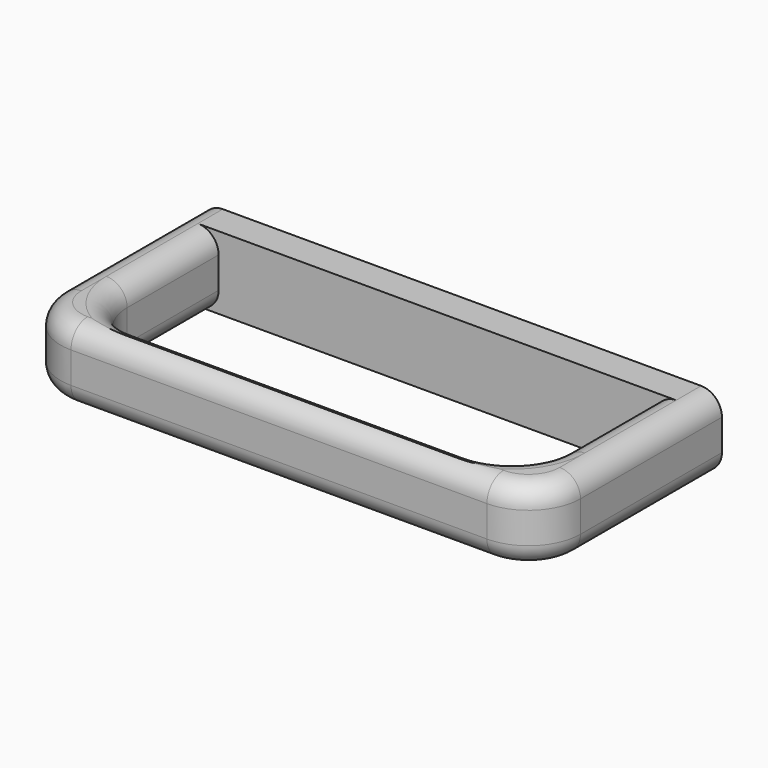
from build123d import *

# Parameters (mm, degrees)
F1_DEPTH     = 7
F2_T1_DEPTH  = 32
F2_T3_DEPTH  = 40
F2_T5_DEPTH  = 22
F2_T7_DEPTH  = 11
F2_T10_ANGLE = 90
F2_T12_ANGLE = 90
F2_T14_ANGLE = 90
F2_T16_ANGLE = 90
F2_T18_ANGLE = 90
F2_T20_ANGLE = 90
F2_T22_ANGLE = 90
F2_T24_ANGLE = 90


# Not quite as in the source:
# - a fillet or chamfer that OpenCascade refuses, or shapes differently, is made with other operations: its cross-section is extruded or revolved along the edge and cut away or added


with BuildPart() as f1:
    # F0 (on Top) → F1 (new body)
    with BuildSketch(Plane.XY):
        with BuildLine():
            Line((-4.4512270018, -28.9949133558), (-54.4512270018, -28.9949133558))
            Line((-54.4512270018, -28.9949133558), (-54.4512270018, -45.9949133558))
            ThreePointArc((-54.4512270018, -45.9949133558), (-52.9867609078, -49.5304472618), (-49.4512270018, -50.9949133558))
            Line((-49.4512270018, -50.9949133558), (-9.4512270018, -50.9949133558))
            ThreePointArc((-9.4512270018, -50.9949133558), (-5.9156930959, -49.5304472618), (-4.4512270018, -45.9949133558))
            Line((-4.4512270018, -45.9949133558), (-4.4512270018, -28.9949133558))
        make_face()
        with BuildLine():
            Line((-50.4512270018, -42.9949133558), (-50.4512270018, -31.9949133558))
            Line((-50.4512270018, -31.9949133558), (-8.4512270018, -31.9949133558))
            Line((-8.4512270018, -31.9949133558), (-8.4512270018, -42.9949133558))
            ThreePointArc((-8.4512270018, -42.9949133558), (-9.9156930959, -46.5304472618), (-13.4512270018, -47.9949133558))
            Line((-13.4512270018, -47.9949133558), (-45.4512270018, -47.9949133558))
            ThreePointArc((-45.4512270018, -47.9949133558), (-48.9867609078, -46.5304472618), (-50.4512270018, -42.9949133558))
        make_face(mode=Mode.SUBTRACT)
    extrude(amount=F1_DEPTH)

    # F2: fillet of radius 2 on 4 edges, made by hand

    # F2_s2 → F2_t1 (cut)
    with BuildSketch(Plane.YZ.offset(-45.4512270018)):
        with BuildLine():
            ThreePointArc((-47.9949133558, 5), (-48.5806997934, 6.4142135624), (-49.9949133558, 7))
            Line((-49.9949133558, 7), (-47.9949133558, 7))
            Line((-47.9949133558, 7), (-47.9949133558, 5))
        make_face()
        with BuildLine():
            ThreePointArc((-47.9949133558, 2), (-48.5806997934, 0.5857864376), (-49.9949133558, 0))
            Line((-49.9949133558, 0), (-47.9949133558, 0))
            Line((-47.9949133558, 0), (-47.9949133558, 2))
        make_face()
    extrude(amount=F2_T1_DEPTH, mode=Mode.SUBTRACT)

    # F2_s4 → F2_t3 (cut)
    with BuildSketch(Plane.YZ.offset(-49.4512270018)):
        with BuildLine():
            ThreePointArc((-50.9949133558, 5), (-50.4091269182, 6.4142135624), (-48.9949133558, 7))
            Line((-48.9949133558, 7), (-50.9949133558, 7))
            Line((-50.9949133558, 7), (-50.9949133558, 5))
        make_face()
        with BuildLine():
            ThreePointArc((-50.9949133558, 2), (-50.4091269182, 0.5857864376), (-48.9949133558, 0))
            Line((-48.9949133558, 0), (-50.9949133558, 0))
            Line((-50.9949133558, 0), (-50.9949133558, 2))
        make_face()
    extrude(amount=F2_T3_DEPTH, mode=Mode.SUBTRACT)

    # F2_s6 → F2_t5 (cut)
    with BuildSketch(Plane.XZ.offset(23.9949133558)):
        with BuildLine():
            ThreePointArc((-54.4512270018, 2), (-53.8654405642, 0.5857864376), (-52.4512270018, 0))
            Line((-52.4512270018, 0), (-54.4512270018, 0))
            Line((-54.4512270018, 0), (-54.4512270018, 2))
        make_face()
        with BuildLine():
            ThreePointArc((-4.4512270018, 2), (-5.0370134395, 0.5857864376), (-6.4512270018, 0))
            Line((-6.4512270018, 0), (-4.4512270018, 0))
            Line((-4.4512270018, 0), (-4.4512270018, 2))
        make_face()
        with BuildLine():
            ThreePointArc((-4.4512270018, 5), (-5.0370134395, 6.4142135624), (-6.4512270018, 7))
            Line((-6.4512270018, 7), (-4.4512270018, 7))
            Line((-4.4512270018, 7), (-4.4512270018, 5))
        make_face()
        with BuildLine():
            ThreePointArc((-54.4512270018, 5), (-53.8654405642, 6.4142135624), (-52.4512270018, 7))
            Line((-52.4512270018, 7), (-54.4512270018, 7))
            Line((-54.4512270018, 7), (-54.4512270018, 5))
        make_face()
    extrude(amount=F2_T5_DEPTH, mode=Mode.SUBTRACT)

    # F2_s8 → F2_t7 (cut)
    with BuildSketch(Plane.XZ.offset(31.9949133558)):
        with BuildLine():
            ThreePointArc((-50.4512270018, 2), (-51.0370134395, 0.5857864376), (-52.4512270018, 0))
            Line((-52.4512270018, 0), (-50.4512270018, 0))
            Line((-50.4512270018, 0), (-50.4512270018, 2))
        make_face()
        with BuildLine():
            ThreePointArc((-8.4512270018, 2), (-7.8654405642, 0.5857864376), (-6.4512270018, 0))
            Line((-6.4512270018, 0), (-8.4512270018, 0))
            Line((-8.4512270018, 0), (-8.4512270018, 2))
        make_face()
        with BuildLine():
            ThreePointArc((-50.4512270018, 5), (-51.0370134395, 6.4142135624), (-52.4512270018, 7))
            Line((-52.4512270018, 7), (-50.4512270018, 7))
            Line((-50.4512270018, 7), (-50.4512270018, 5))
        make_face()
        with BuildLine():
            ThreePointArc((-8.4512270018, 5), (-7.8654405642, 6.4142135624), (-6.4512270018, 7))
            Line((-6.4512270018, 7), (-8.4512270018, 7))
            Line((-8.4512270018, 7), (-8.4512270018, 5))
        make_face()
    extrude(amount=F2_T7_DEPTH, mode=Mode.SUBTRACT)

    # F2_s9 → F2_t10 (revolve, cut)
    with BuildSketch(Plane.XZ.offset(42.9949133558)):
        with BuildLine():
            ThreePointArc((-8.4512270018, 2), (-7.8654405642, 0.5857864376), (-6.4512270018, 0))
            Line((-6.4512270018, 0), (-8.4512270018, 0))
            Line((-8.4512270018, 0), (-8.4512270018, 2))
        make_face()
    revolve(axis=Axis((-13.4512270018, -42.9949133558, 0), (0, 0, -1)), revolution_arc=F2_T10_ANGLE, mode=Mode.SUBTRACT)

    # F2_s11 → F2_t12 (revolve, cut)
    with BuildSketch(Plane.YZ.offset(-45.4512270018)):
        with BuildLine():
            ThreePointArc((-47.9949133558, 2), (-48.5806997934, 0.5857864376), (-49.9949133558, 0))
            Line((-49.9949133558, 0), (-47.9949133558, 0))
            Line((-47.9949133558, 0), (-47.9949133558, 2))
        make_face()
    revolve(axis=Axis((-45.4512270018, -42.9949133558, 0), (0, 0, -1)), revolution_arc=F2_T12_ANGLE, mode=Mode.SUBTRACT)

    # F2_s13 → F2_t14 (revolve, cut)
    with BuildSketch(Plane.XZ.offset(45.9949133558)):
        with BuildLine():
            ThreePointArc((-54.4512270018, 2), (-53.8654405642, 0.5857864376), (-52.4512270018, 0))
            Line((-52.4512270018, 0), (-54.4512270018, 0))
            Line((-54.4512270018, 0), (-54.4512270018, 2))
        make_face()
    revolve(axis=Axis((-49.4512270018, -45.9949133558, 0), (0, 0, 1)), revolution_arc=F2_T14_ANGLE, mode=Mode.SUBTRACT)

    # F2_s15 → F2_t16 (revolve, cut)
    with BuildSketch(Plane.YZ.offset(-9.4512270018)):
        with BuildLine():
            ThreePointArc((-50.9949133558, 2), (-50.4091269182, 0.5857864376), (-48.9949133558, 0))
            Line((-48.9949133558, 0), (-50.9949133558, 0))
            Line((-50.9949133558, 0), (-50.9949133558, 2))
        make_face()
    revolve(axis=Axis((-9.4512270018, -45.9949133558, 0), (0, 0, 1)), revolution_arc=F2_T16_ANGLE, mode=Mode.SUBTRACT)

    # F2_s17 → F2_t18 (revolve, cut)
    with BuildSketch(Plane.XZ.offset(45.9949133558)):
        with BuildLine():
            ThreePointArc((-54.4512270018, 5), (-53.8654405642, 6.4142135624), (-52.4512270018, 7))
            Line((-52.4512270018, 7), (-54.4512270018, 7))
            Line((-54.4512270018, 7), (-54.4512270018, 5))
        make_face()
    revolve(axis=Axis((-49.4512270018, -45.9949133558, 7), (0, 0, 1)), revolution_arc=F2_T18_ANGLE, mode=Mode.SUBTRACT)

    # F2_s19 → F2_t20 (revolve, cut)
    with BuildSketch(Plane.YZ.offset(-9.4512270018)):
        with BuildLine():
            ThreePointArc((-50.9949133558, 5), (-50.4091269182, 6.4142135624), (-48.9949133558, 7))
            Line((-48.9949133558, 7), (-50.9949133558, 7))
            Line((-50.9949133558, 7), (-50.9949133558, 5))
        make_face()
    revolve(axis=Axis((-9.4512270018, -45.9949133558, 7), (0, 0, 1)), revolution_arc=F2_T20_ANGLE, mode=Mode.SUBTRACT)

    # F2_s21 → F2_t22 (revolve, cut)
    with BuildSketch(Plane.XZ.offset(42.9949133558)):
        with BuildLine():
            ThreePointArc((-8.4512270018, 5), (-7.8654405642, 6.4142135624), (-6.4512270018, 7))
            Line((-6.4512270018, 7), (-8.4512270018, 7))
            Line((-8.4512270018, 7), (-8.4512270018, 5))
        make_face()
    revolve(axis=Axis((-13.4512270018, -42.9949133558, 7), (0, 0, -1)), revolution_arc=F2_T22_ANGLE, mode=Mode.SUBTRACT)

    # F2_s23 → F2_t24 (revolve, cut)
    with BuildSketch(Plane.YZ.offset(-45.4512270018)):
        with BuildLine():
            ThreePointArc((-47.9949133558, 5), (-48.5806997934, 6.4142135624), (-49.9949133558, 7))
            Line((-49.9949133558, 7), (-47.9949133558, 7))
            Line((-47.9949133558, 7), (-47.9949133558, 5))
        make_face()
    revolve(axis=Axis((-45.4512270018, -42.9949133558, 7), (0, 0, -1)), revolution_arc=F2_T24_ANGLE, mode=Mode.SUBTRACT)


solid = f1.part
